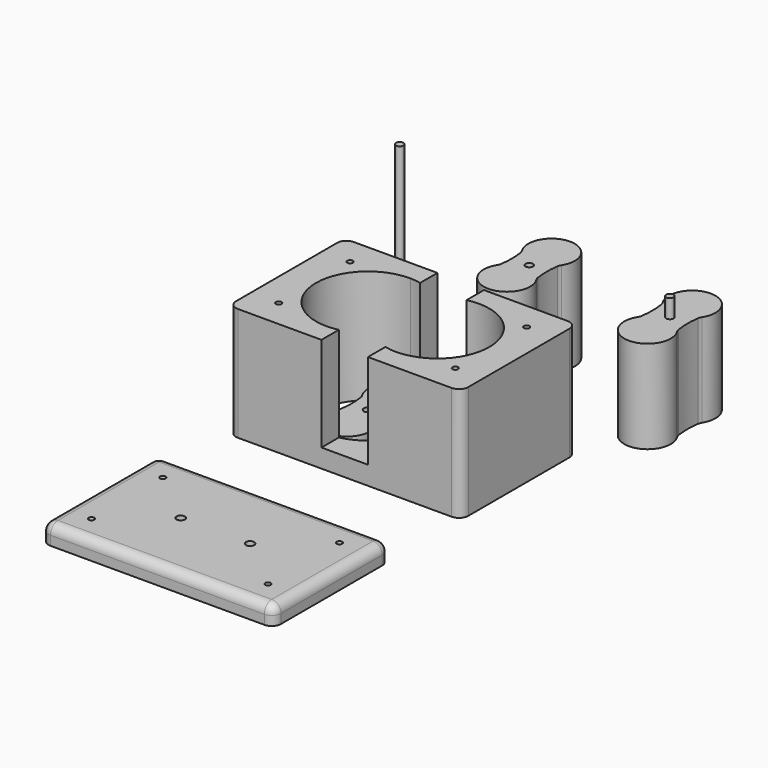
from build123d import *

# Parameters (mm, degrees)
F0_R         = 2
F1_DEPTH     = 50
F2_DEPTH     = 60
F3_R         = 5
F3_2_R       = 5
F0_R_2       = 2.25
F4_DEPTH     = 10
F0_W         = 125
F0_H         = 78
F0_R_3       = 1.5
F5_DEPTH     = 61
F6_DEPTH     = 100
F7_R         = 5
F8_T1_DEPTH  = 17.5
F8_S5_W      = 5
F8_S5_H      = 5
F8_T6_DEPTH  = 5
F8_S11_W     = 5
F8_S11_H     = 5
F8_T12_DEPTH = 5
F8_S17_W     = 5
F8_S17_H     = 5
F8_T18_DEPTH = 5
F8_S23_W     = 5
F8_S23_H     = 5
F8_T24_DEPTH = 5
F9_R         = 5


# Not quite as in the source:
# - a fillet or chamfer that OpenCascade refuses, or shapes differently, is made with other operations: its cross-section is extruded or revolved along the edge and cut away or added


with BuildPart() as f1:
    # F0 (on Top) → F1 (new body)
    with BuildSketch(Plane.XY):
        with BuildLine():
            ThreePointArc((-10.1040010514, 7.6407090862), (-9.4250014394, 0.0038853003), (-10.0986804598, -7.6334096781))
            ThreePointArc((-10.0986804598, -7.6334096781), (0, -27.5), (10.0986804598, -7.6334096781))
            ThreePointArc((10.0986804598, -7.6334096781), (9.4248676238, 0), (10.0986804598, 7.6334096781))
            ThreePointArc((10.0986804598, 7.6334096781), (0.0045163606, 27.4999991841), (-10.1040010514, 7.6407090862))
        make_face()
        Circle(F0_R, mode=Mode.SUBTRACT)
    extrude(amount=F1_DEPTH)

    # F3
    f3_edges = [f1.edges().sort_by_distance(p)[0] for p in [
        (10.09868, 7.63341, 25),
        (10.09868, -7.63341, 25),
        (-10.09868, -7.63341, 25),
        (-10.104001, 7.640709, 25),
    ]]
    fillet(f3_edges, radius=F3_R)


with BuildPart() as f1b:
    # F0 (on Top) → F1, piece 2 (new body)
    with BuildSketch(Plane.XY):
        with BuildLine():
            ThreePointArc((65.5496659632, 7.651961291), (66.2286655751, 0.0151375051), (65.5549865547, -7.6221574733))
            ThreePointArc((65.5549865547, -7.6221574733), (75.6536670145, -27.4887477952), (85.7523474743, -7.6221574733))
            ThreePointArc((85.7523474743, -7.6221574733), (85.0785346383, 0.0112522048), (85.7523474743, 7.644661883))
            ThreePointArc((85.7523474743, 7.644661883), (75.6581833751, 27.5112513889), (65.5496659632, 7.651961291))
        make_face()
        with Locations((75.6536670145, 0)):
            Circle(F0_R, mode=Mode.SUBTRACT)
    extrude(amount=F1_DEPTH)

    # F0 (on Top) → F2 (join)
    with BuildSketch(Plane.XY):
        with Locations((75.6536670145, 0)):
            Circle(F0_R)
    extrude(amount=F2_DEPTH)

    # F3#2
    f3_2_edges = [f1b.edges().sort_by_distance(p)[0] for p in [
        (85.752347, -7.622157, 25),
        (85.752347, 7.644662, 25),
        (65.554987, -7.622157, 25),
        (65.549666, 7.651961, 25),
    ]]
    fillet(f3_2_edges, radius=F3_2_R)


with BuildPart() as f4:
    # F0 (on Top) → F4 (new body)
    with BuildSketch(Plane.XY):
        with BuildLine():
            ThreePointArc((-5.6864082098, -98.9216233409), (-9.3439997167, -85.1549598907), (-5.755221033, -71.3701978056))
            ThreePointArc((-5.755221033, -71.3701978056), (-8.7770088894, -61.5327286758), (-18.1557578595, -57.2964486466))
            ThreePointArc((-18.1557578595, -57.2964486466), (-29.2966989423, -64.1281656801), (-28.2597589108, -77.1557395604))
            ThreePointArc((-28.2597589108, -77.1557395604), (-27.5807592988, -84.7925633463), (-28.2544383193, -92.4298583247))
            ThreePointArc((-28.2544383193, -92.4298583247), (-29.2987462159, -105.4607059226), (-18.1557578595, -112.2964486466))
            ThreePointArc((-18.1557578595, -112.2964486466), (-9.012855795, -108.320376253), (-5.6864082098, -98.9216233409))
        make_face()
        with Locations((-18.6559129506, -85.0850269198)):
            Circle(F0_R_2, mode=Mode.SUBTRACT)
    extrude(amount=F4_DEPTH)


with BuildPart() as f4b:
    # F0 (on Top) → F4, piece 2 (new body)
    with BuildSketch(Plane.XY):
        with BuildLine():
            ThreePointArc((9.3440870494, -85.0850269198), (6.9015278702, -73.6474914033), (0, -64.2054456985))
            ThreePointArc((0, -64.2054456985), (-3.1735637059, -67.5500918215), (-5.755221033, -71.3701978056))
            ThreePointArc((-5.755221033, -71.3701978056), (-6.5375962311, -74.408207571), (-8.0517568081, -77.1557395604))
            ThreePointArc((-8.0517568081, -77.1557395604), (-8.7288795316, -84.7925640001), (-8.0570773996, -92.4298583247))
            ThreePointArc((-8.0570773996, -92.4298583247), (-6.4141758105, -95.5086460639), (-5.6864082098, -98.9216233409))
            ThreePointArc((-5.6864082098, -98.9216233409), (-3.1297002584, -102.6744287604), (0, -105.9646081412))
            ThreePointArc((0, -105.9646081412), (6.9015278702, -96.5225624363), (9.3440870494, -85.0850269198))
        make_face()
        with BuildLine():
            ThreePointArc((12.5, -112.3999447441), (36.1435433988, -106.9524177406), (46.6559129506, -85.0850269198))
            ThreePointArc((46.6559129506, -85.0850269198), (36.1435433988, -63.2176360991), (12.5, -57.7701090956))
            ThreePointArc((12.5, -57.7701090956), (5.8395146486, -60.1904505113), (0, -64.2054456985))
            ThreePointArc((0, -64.2054456985), (6.9015278702, -73.6474914033), (9.3440870494, -85.0850269198))
            ThreePointArc((9.3440870494, -85.0850269198), (6.9015278702, -96.5225624363), (0, -105.9646081412))
            ThreePointArc((0, -105.9646081412), (5.8395146486, -109.9796033284), (12.5, -112.3999447441))
        make_face()
        with Locations((18.6559129506, -85.0850269198)):
            Circle(F0_R_2, mode=Mode.SUBTRACT)
        with BuildLine():
            Line((12.5, -124.0850269198), (12.5, -112.3999447441))
            ThreePointArc((12.5, -112.3999447441), (5.8395146486, -109.9796033284), (0, -105.9646081412))
            ThreePointArc((0, -105.9646081412), (-5.8395146486, -109.9796033284), (-12.5, -112.3999447441))
            Line((-12.5, -112.3999447441), (-12.5, -124.0850269198))
            Line((-12.5, -124.0850269198), (12.5, -124.0850269198))
        make_face()
        with BuildLine():
            ThreePointArc((0, -64.2054456985), (5.8395146486, -60.1904505113), (12.5, -57.7701090956))
            Line((12.5, -57.7701090956), (12.5, -46.0850269198))
            Line((12.5, -46.0850269198), (-12.5, -46.0850269198))
            Line((-12.5, -46.0850269198), (-12.5, -57.7701090956))
            ThreePointArc((-12.5, -57.7701090956), (-5.8395146486, -60.1904505113), (0, -64.2054456985))
        make_face()
    extrude(amount=F4_DEPTH)

    # F0 (on Top) → F5 (join)
    with BuildSketch(Plane.XY):
        with BuildLine():
            ThreePointArc((-18.1557578595, -57.0894943319), (-15.3105251467, -57.2855956228), (-12.5, -57.7701090956))
            Line((-12.5, -57.7701090956), (-12.5, -46.0850269198))
            Line((-12.5, -46.0850269198), (-62.5, -46.0850269198))
            Line((-62.5, -46.0850269198), (-62.5, -124.0850269198))
            Line((-62.5, -124.0850269198), (-12.5, -124.0850269198))
            Line((-12.5, -124.0850269198), (-12.5, -112.3999447441))
            ThreePointArc((-12.5, -112.3999447441), (-15.3105251467, -112.8844582169), (-18.1557578595, -113.0805595078))
            ThreePointArc((-18.1557578595, -113.0805595078), (-46.6559129506, -85.0850269198), (-18.1557578595, -57.0894943319))
        make_face()
        with Locations((-47.5, -109.0850269198)):
            Circle(F0_R_3, mode=Mode.SUBTRACT)
        with Locations((-47.5, -61.0850269198)):
            Circle(F0_R_3, mode=Mode.SUBTRACT)
        with BuildLine():
            ThreePointArc((12.5, -57.7701090956), (36.1435433988, -63.2176360991), (46.6559129506, -85.0850269198))
            ThreePointArc((46.6559129506, -85.0850269198), (36.1435433988, -106.9524177406), (12.5, -112.3999447441))
            Line((12.5, -112.3999447441), (12.5, -124.0850269198))
            Line((12.5, -124.0850269198), (62.5, -124.0850269198))
            Line((62.5, -124.0850269198), (62.5, -46.0850269198))
            Line((62.5, -46.0850269198), (12.5, -46.0850269198))
            Line((12.5, -46.0850269198), (12.5, -57.7701090956))
        make_face()
        with Locations((47.5, -109.0850269198)):
            Circle(F0_R_3, mode=Mode.SUBTRACT)
        with Locations((47.5, -61.0850269198)):
            Circle(F0_R_3, mode=Mode.SUBTRACT)
    extrude(amount=F5_DEPTH)

    # F9
    f9_edges = [f4b.edges().sort_by_distance(p)[0] for p in [
        (-62.5, -46.085027, 30.5),
        (-62.5, -124.085027, 30.5),
        (62.5, -46.085027, 30.5),
        (62.5, -124.085027, 30.5),
    ]]
    fillet(f9_edges, radius=F9_R)


with BuildPart() as f4c:
    # F0 (on Top) → F4, piece 3 (new body)
    with BuildSketch(Plane.XY):
        with Locations((0, -211.0378489494)):
            Rectangle(F0_W, F0_H)
        with Locations((-47.5, -235.0378489494)):
            Circle(F0_R_3, mode=Mode.SUBTRACT)
        with Locations((-47.5, -187.0378489494)):
            Circle(F0_R_3, mode=Mode.SUBTRACT)
        with Locations((-18.6559129506, -211.0378489494)):
            Circle(F0_R_2, mode=Mode.SUBTRACT)
        with Locations((47.5, -235.0378489494)):
            Circle(F0_R_3, mode=Mode.SUBTRACT)
        with Locations((18.6559129506, -211.0378489494)):
            Circle(F0_R_2, mode=Mode.SUBTRACT)
        with Locations((47.5, -187.0378489494)):
            Circle(F0_R_3, mode=Mode.SUBTRACT)
    extrude(amount=F4_DEPTH)

    # F7
    f7_edges = [f4c.edges().sort_by_distance(p)[0] for p in [
        (-62.5, -211.037849, 10),
        (0, -172.037849, 10),
        (0, -250.037849, 10),
        (62.5, -211.037849, 10),
    ]]
    fillet(f7_edges, radius=F7_R)

    # F8: fillet of radius 5 on 4 edges, made by hand

    # F8_s2 → F8_t1 (cut)
    with BuildSketch(Plane.XY.offset(-12.5)):
        with BuildLine():
            ThreePointArc((57.5, -172.0378489494), (61.0355339059, -173.5023150435), (62.5, -177.0378489494))
            Line((62.5, -177.0378489494), (62.5, -172.0378489494))
            Line((62.5, -172.0378489494), (57.5, -172.0378489494))
        make_face()
        with BuildLine():
            ThreePointArc((57.5, -250.0378489494), (61.0355339059, -248.5733828554), (62.5, -245.0378489494))
            Line((62.5, -245.0378489494), (62.5, -250.0378489494))
            Line((62.5, -250.0378489494), (57.5, -250.0378489494))
        make_face()
        with BuildLine():
            ThreePointArc((-62.5, -245.0378489494), (-61.0355339059, -248.5733828554), (-57.5, -250.0378489494))
            Line((-57.5, -250.0378489494), (-62.5, -250.0378489494))
            Line((-62.5, -250.0378489494), (-62.5, -245.0378489494))
        make_face()
        with BuildLine():
            ThreePointArc((-62.5, -177.0378489494), (-61.0355339059, -173.5023150435), (-57.5, -172.0378489494))
            Line((-57.5, -172.0378489494), (-62.5, -172.0378489494))
            Line((-62.5, -172.0378489494), (-62.5, -177.0378489494))
        make_face()
    extrude(amount=F8_T1_DEPTH, mode=Mode.SUBTRACT)


with BuildPart() as f6:
    # F0 (on Top) → F6 (new body)
    with BuildSketch(Plane.XY):
        with Locations((-51.2222014368, -23.0306889862)):
            Circle(F0_R)
    extrude(amount=F6_DEPTH)


with BuildPart() as f8_tool4:
    # F8_s5 → F8_t6 (new body)
    with BuildSketch(Plane.YZ.offset(-57.5)):
        with Locations((-174.5378489494, 7.5)):
            Rectangle(F8_S5_W, F8_S5_H)
    extrude(amount=-F8_T6_DEPTH)

    # F8_s7 → F8_t8 (revolve, cut)
    with BuildSketch(Plane(origin=(-57.5, -177.0378489494, 5), x_dir=(0, -0.7071067812, -0.7071067812), z_dir=(0, 0.7071067812, -0.7071067812))):
        with BuildLine():
            ThreePointArc((0, -5), (5, 0), (0, 5))
            Line((0, 5), (0, -5))
        make_face()
    revolve(axis=Axis((-57.5, -177.0378489494, 5), (-1, 0, 0)), mode=Mode.SUBTRACT)


with BuildPart() as f4c_1:
    add(f4c.part)

    # F8_t3: cut F8_tool4
    add(f8_tool4.part, mode=Mode.SUBTRACT)


with BuildPart() as f8_tool10:
    # F8_s11 → F8_t12 (new body)
    with BuildSketch(Plane.YZ.offset(-57.5)):
        with Locations((-247.5378489494, 7.5)):
            Rectangle(F8_S11_W, F8_S11_H)
    extrude(amount=-F8_T12_DEPTH)

    # F8_s13 → F8_t14 (revolve, cut)
    with BuildSketch(Plane(origin=(-57.5, -245.0378489494, 5), x_dir=(0, 0.7071067812, -0.7071067812), z_dir=(0, 0.7071067812, 0.7071067812))):
        with BuildLine():
            ThreePointArc((0, -5), (5, 0), (0, 5))
            Line((0, 5), (0, -5))
        make_face()
    revolve(axis=Axis((-57.5, -245.0378489494, 5), (-1, 0, 0)), mode=Mode.SUBTRACT)


with BuildPart() as f4c_2:
    add(f4c_1.part)

    # F8_t9: cut F8_tool10
    add(f8_tool10.part, mode=Mode.SUBTRACT)


with BuildPart() as f8_tool16:
    # F8_s17 → F8_t18 (new body)
    with BuildSketch(Plane.XZ.offset(245.0378489494)):
        with Locations((60, 7.5)):
            Rectangle(F8_S17_W, F8_S17_H)
    extrude(amount=F8_T18_DEPTH)

    # F8_s19 → F8_t20 (revolve, cut)
    with BuildSketch(Plane(origin=(57.5, -245.0378489494, 5), x_dir=(-0.7071067812, 0, -0.7071067812), z_dir=(-0.7071067812, 0, 0.7071067812))):
        with BuildLine():
            ThreePointArc((0, -5), (5, 0), (0, 5))
            Line((0, 5), (0, -5))
        make_face()
    revolve(axis=Axis((57.5, -245.0378489494, 5), (0, -1, 0)), mode=Mode.SUBTRACT)


with BuildPart() as f4c_3:
    add(f4c_2.part)

    # F8_t15: cut F8_tool16
    add(f8_tool16.part, mode=Mode.SUBTRACT)


with BuildPart() as f8_tool22:
    # F8_s23 → F8_t24 (new body)
    with BuildSketch(Plane.XZ.offset(177.0378489494)):
        with Locations((60, 7.5)):
            Rectangle(F8_S23_W, F8_S23_H)
    extrude(amount=-F8_T24_DEPTH)

    # F8_s25 → F8_t26 (revolve, cut)
    with BuildSketch(Plane(origin=(57.5, -177.0378489494, 5), x_dir=(-0.7071067812, 0, -0.7071067812), z_dir=(0.7071067812, 0, -0.7071067812))):
        with BuildLine():
            ThreePointArc((0, -5), (5, 0), (0, 5))
            Line((0, 5), (0, -5))
        make_face()
    revolve(axis=Axis((57.5, -177.0378489494, 5), (0, 1, 0)), mode=Mode.SUBTRACT)


with BuildPart() as f4c_4:
    add(f4c_3.part)

    # F8_t21: cut F8_tool22
    add(f8_tool22.part, mode=Mode.SUBTRACT)


solid = Compound([f1.part, f1b.part, f4.part, f4b.part, f6.part, f4c_4.part])
